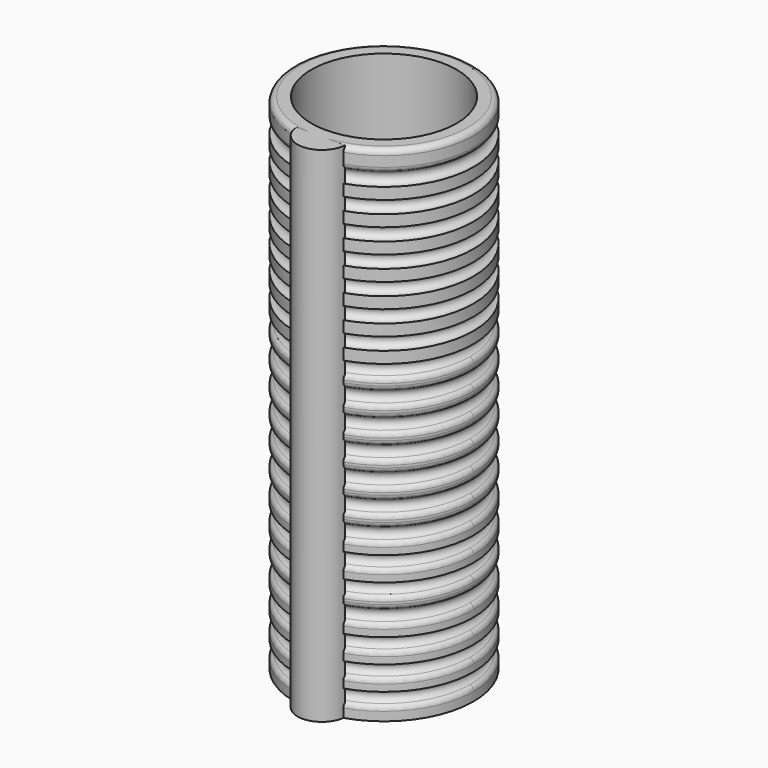
from build123d import *

# Parameters (mm, degrees)
F0_R      = 16
F0_R_2    = 13
F1_DEPTH  = 90
F3_DEPTH  = 25
F0_R_3    = 5.95
F0_R_4    = 3.95
F4_DEPTH  = 25
F5_DEPTH  = 100.3
F7_R      = 1.1303713172
F9_R      = 1
F11_DEPTH = 90


with BuildPart() as f1:
    # F0 (on Top) → F1 (new body)
    with BuildSketch(Plane.XY):
        Circle(F0_R)
        Circle(F0_R_2, mode=Mode.SUBTRACT)
    extrude(amount=F1_DEPTH)

    # F2 (on Top) → F3 (join)
    with BuildSketch(Plane.XY):
        Polygon((-2.6178282159, -1.5114038251), (0, 0), (-14.5057244226, 0), (-14.5057244226, -3.0228076503), (-1.7452188106, -3.0228076503), align=None)
        Polygon((-2.6178282159, 1.5114038251), (0, 0), (0, 3.0228076503), (-1.7452188106, 3.0228076503), align=None)
        Polygon((7.2528622113, -12.5623258503), (0, 0), (0, -3.0228076503), (-1.7452188106, -3.0228076503), (4.6350339954, -14.0737296754), align=None)
        Polygon((2.6178282159, -1.5114038251), (0, 0), (7.2528622113, -12.5623258503), (9.8706904272, -11.0509220252), (3.4904376212, 0), align=None)
        Polygon((7.2528622113, 12.5623258503), (0, 0), (2.6178282159, 1.5114038251), (3.4904376212, 0), (9.8706904272, 11.0509220252), align=None)
        Polygon((0, -3.0228076503), (0, 0), (-2.6178282159, -1.5114038251), (-1.7452188106, -3.0228076503), align=None)
        Polygon((0, 3.0228076503), (0, 0), (7.2528622113, 12.5623258503), (4.6350339954, 14.0737296754), (-1.7452188106, 3.0228076503), align=None)
        Polygon((-14.5057244226, 0), (0, 0), (-2.6178282159, 1.5114038251), (-1.7452188106, 3.0228076503), (-14.5057244226, 3.0228076503), align=None)
        Polygon((2.6178282159, 1.5114038251), (0, 0), (2.6178282159, -1.5114038251), (3.4904376212, 0), align=None)
    extrude(amount=F3_DEPTH)

    # F0 (on Top) → F4 (join)
    with BuildSketch(Plane.XY):
        Circle(F0_R_3)
        Circle(F0_R_4, mode=Mode.SUBTRACT)
        Circle(F0_R_4)
    extrude(amount=F4_DEPTH)

    # F0 (on Top) → F5 (cut)
    with BuildSketch(Plane.XY):
        Circle(F0_R_4)
    extrude(amount=F5_DEPTH, mode=Mode.SUBTRACT)

    # F7 (on Front) → F8 (revolve, cut)
    with BuildSketch(Plane.XZ):
        with Locations((15.8607251942, 3.5246065818)):
            Circle(F7_R)
        with Locations((15.8607251942, 7.8246065818)):
            Circle(F7_R)
        with Locations((15.8607251942, 12.1246065818)):
            Circle(F7_R)
        with Locations((15.8607251942, 16.4246065818)):
            Circle(F7_R)
        with Locations((15.8607251942, 20.7246065818)):
            Circle(F7_R)
        with Locations((15.8607251942, 25.0246065818)):
            Circle(F7_R)
        with Locations((15.8607251942, 29.3246065818)):
            Circle(F7_R)
        with Locations((15.8607251942, 33.6246065818)):
            Circle(F7_R)
        with Locations((15.8607251942, 37.9246065818)):
            Circle(F7_R)
        with Locations((15.8607251942, 42.2246065818)):
            Circle(F7_R)
        with Locations((15.8607251942, 46.5246065818)):
            Circle(F7_R)
        with Locations((15.8607251942, 50.8246065818)):
            Circle(F7_R)
        with Locations((15.8607251942, 55.1246065818)):
            Circle(F7_R)
        with Locations((15.8607251942, 59.4246065818)):
            Circle(F7_R)
        with Locations((15.8607251942, 63.7246065818)):
            Circle(F7_R)
        with Locations((15.8607251942, 68.0246065818)):
            Circle(F7_R)
        with Locations((15.8607251942, 72.3246065818)):
            Circle(F7_R)
        with Locations((15.8607251942, 76.6246065818)):
            Circle(F7_R)
        with Locations((15.8607251942, 80.9246065818)):
            Circle(F7_R)
        with Locations((15.8607251942, 85.2246065818)):
            Circle(F7_R)
    revolve(axis=Axis((0, 0, 23.4791748226), (0, 0, -1)), mode=Mode.SUBTRACT)

    # F9
    f9_edges = [f1.edges().sort_by_distance(p)[0] for p in [
        (-16, 0, 43.346365),
        (16, 0, 44.374607),
        (-16, 0, 45.402848),
        (-16, 0, 17.546365),
        (16, 0, 18.574607),
        (-16, 0, 19.602848),
        (-16, 0, 39.046365),
        (16, 0, 40.074607),
        (-16, 0, 41.102848),
        (-16, 0, 47.646365),
        (16, 0, 48.674607),
        (-16, 0, 49.702848),
        (-16, 0, 51.946365),
        (16, 0, 52.974607),
        (-16, 0, 54.002848),
        (-16, 0, 2.402848),
        (-16, 0, 6.702848),
        (-16, 0, 90),
        (-16, 0, 86.346365),
        (-16, 0, 11.002848),
        (-16, 0, 15.302848),
        (-16, 0, 23.902848),
        (-16, 0, 28.202848),
        (-16, 0, 30.446365),
        (-16, 0, 32.502848),
        (-16, 0, 34.746365),
        (-16, 0, 36.802848),
    ]]
    fillet(f9_edges, radius=F9_R)

    # F10 (on Top) → F11 (join, through all)
    with BuildSketch(Plane.XY):
        with BuildLine():
            Line((4.9498842896, -14.8996980861), (-3.7427230272, -14.8996980861))
            ThreePointArc((-3.7427230272, -14.8996980861), (0.6035806312, -18.9899925898), (4.9498842896, -14.8996980861))
        make_face()
    extrude(amount=F11_DEPTH)


solid = f1.part
